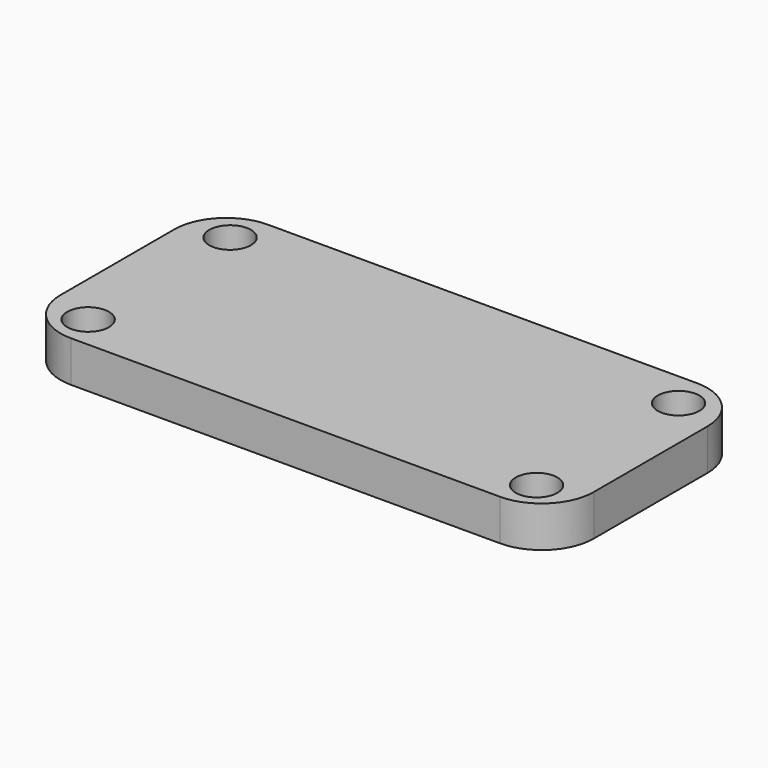
from build123d import *

# Parameters (mm, degrees)
F1_DEPTH = 4.99999
F2_R     = 2.54
F3_DEPTH = 12.7


# Not quite as in the source:
# - the program builds the solid bodies; features that only make, move or delete a surface that nothing else refers to are left out


with BuildPart() as f1:
    # F0 (on Top) → F1 (new body)
    with BuildSketch(Plane.XY):
        with BuildLine():
            Line((24.9985645242, 15.2049488522), (-27.3015594758, 15.2049488522))
            ThreePointArc((-27.3015594758, 15.2049488522), (-31.7916875363, 13.3450769127), (-33.6515594758, 8.8549488522))
            Line((-33.6515594758, 8.8549488522), (-33.6515594758, -8.4449911478))
            ThreePointArc((-33.6515594758, -8.4449911478), (-31.7916875363, -12.9351192083), (-27.3015594758, -14.7949911478))
            Line((-27.3015594758, -14.7949911478), (24.9985645242, -14.7949911478))
            ThreePointArc((24.9985645242, -14.7949911478), (29.4886925847, -12.9351192083), (31.3485645242, -8.4449911478))
            Line((31.3485645242, -8.4449911478), (31.3485645242, 8.8549488522))
            ThreePointArc((31.3485645242, 8.8549488522), (29.4886925847, 13.3450769127), (24.9985645242, 15.2049488522))
        make_face()
    extrude(amount=F1_DEPTH)

    # F2 (on Top) → F3 (cut, symmetric)
    with BuildSketch(Plane.XY):
        with Locations((-28.451833874, 10.8810858801)):
            Circle(F2_R)
        with Locations((-28.451833874, -10.7532069087)):
            Circle(F2_R)
        with Locations((26.2153949589, -10.7532069087)):
            Circle(F2_R)
        with Locations((26.2153949589, 10.8810858801)):
            Circle(F2_R)
    extrude(amount=F3_DEPTH, both=True, mode=Mode.SUBTRACT)


solid = f1.part
